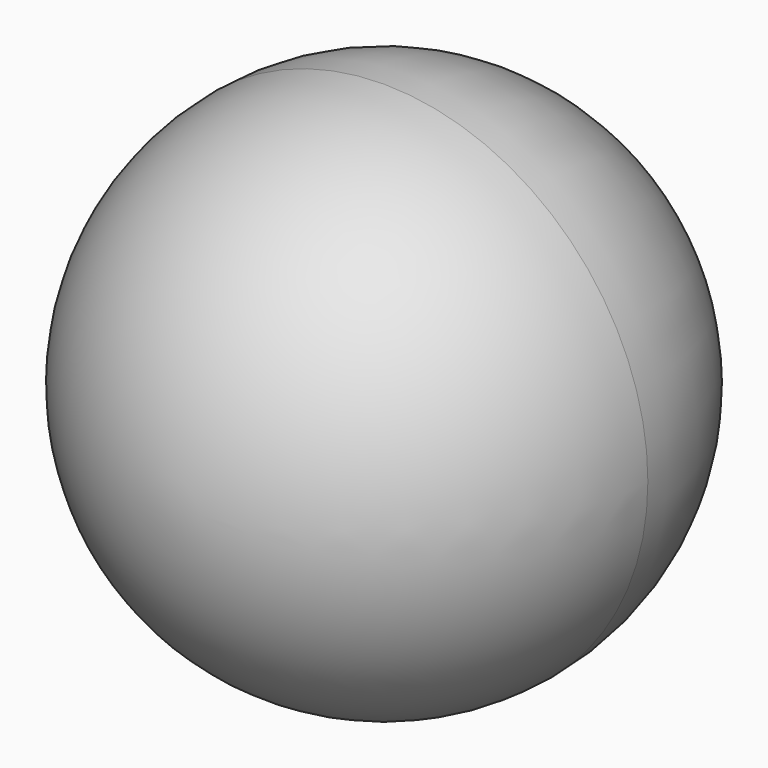
from build123d import *

# Parameters (mm, degrees)
F0_R     = 76.2
F1_DEPTH = 76.2
F2_R     = 76.2
F3_R     = 76.19999


# Not quite as in the source:
# - a fillet or chamfer is up to 0.001 mm smaller than in the source, because OpenCascade refuses the exact size


with BuildPart() as f1:
    # F0 (on Front) → F1 (new body, symmetric)
    with BuildSketch(Plane.XZ):
        Circle(F0_R)
    extrude(amount=F1_DEPTH, both=True)

    # F2
    f2_edges = [f1.edges().sort_by_distance(p)[0] for p in [
        (-76.2, -76.2, 0),
    ]]
    fillet(f2_edges, radius=F2_R)

    # F3 (radius 76.2 in the source; OpenCascade refuses exactly that, so slightly less here)
    f3_edges = [f1.edges().sort_by_distance(p)[0] for p in [
        (-76.2, 76.2, 0),
    ]]
    fillet(f3_edges, radius=F3_R)


solid = f1.part
